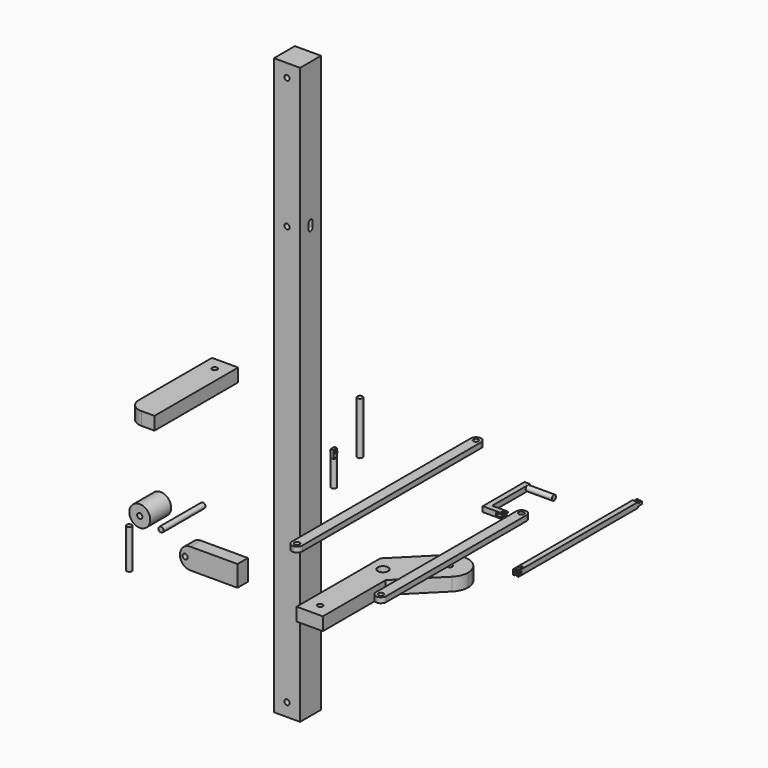
from build123d import *

# Parameters (mm, degrees)
F0_W           = 10
F0_H           = 5
F1_DEPTH       = 40
F2_R           = 5
F3_R           = 1
F4_DEPTH       = 10
F6_DEPTH       = 5
F7_R           = 2
F7_R_2         = 1
F8_DEPTH       = 5.001
F9_R           = 1
F10_DEPTH      = 10
F11_W          = 10
F11_H          = 220
F12_DEPTH      = 10
F13_R          = 1
F14_DEPTH      = 15.1366173212
F15_R          = 1
F16_DEPTH      = 15.1366173212
F17_R          = 1
F18_DEPTH      = 20
F19_W          = 4
F19_H          = 2
F20_DEPTH      = 89.44
F21_R          = 1
F22_DEPTH      = 111.2488439361
F23_R          = 1.99999
F24_W          = 4
F24_H          = 2
F25_DEPTH      = 71.08
F26_R          = 1
F27_DEPTH      = 92.3698075909
F28_R          = 1.99999
F29_W          = 6
F29_H          = 2
F30_DEPTH      = 2
F29_W_2        = 2
F29_H_2        = 57
F31_R          = 1
F32_DEPTH      = 10
F33_R          = 1
F34_DEPTH      = 10
F35_W          = 1
F35_H          = 1.7320508076
F36_DEPTH      = 3
F37_R          = 0.5
F38_DEPTH      = 0.5
F38_DEPTH_BACK = 1.5
F39_W          = 2
F39_H          = 1
F40_DEPTH      = 3
F41_R          = 0.5
F42_DEPTH      = 62.7122059742
F43_W          = 2
F43_H          = 1
F44_DEPTH      = 2
F45_R          = 0.5
F46_DEPTH      = 0.5
F46_DEPTH_BACK = 1.5
F47_W          = 1
F47_H          = 2
F48_DEPTH      = 3
F49_R          = 0.5
F50_DEPTH      = 106.8696667108
F52_DEPTH      = 5
F53_R          = 1
F54_DEPTH      = 76.7775256912
F55_R          = 1
F56_DEPTH      = 20
F57_R          = 4
F57_R_2        = 1
F58_DEPTH      = 10
F60_DEPTH      = 25
F61_R          = 1
F62_DEPTH      = 15


# Not quite as in the source:
# - a fillet or chamfer is up to 0.001 mm smaller than in the source, because OpenCascade refuses the exact size


with BuildPart() as f1:
    # F0 (on Front) → F1 (new body)
    with BuildSketch(Plane.XZ):
        with Locations((-59.1135102832, 41.6379347444)):
            Rectangle(F0_W, F0_H)
    extrude(amount=F1_DEPTH)

    # F2
    f2_edges = [f1.edges().sort_by_distance(p)[0] for p in [
        (-64.11351, -40, 41.637935),
    ]]
    fillet(f2_edges, radius=F2_R)

    # F3 (on face) → F4 (cut)
    with BuildSketch(Plane.XY.offset(44.1379347444)):
        with Locations((-59.1135102832, -5)):
            Circle(F3_R)
    extrude(amount=-F4_DEPTH, mode=Mode.SUBTRACT)


with BuildPart() as f6:
    # F5 (on Top) → F6 (new body)
    with BuildSketch(Plane.XY):
        Polygon((19.0748270126, -21.0775861144), (9.0748270126, -11.0775861144), (9.0748270126, -51.0775861144), (19.0748270126, -51.0775861144), align=None)
        with BuildLine():
            Line((23.2169626363, 3.0645495093), (9.0748270126, -11.0775861144))
            Line((9.0748270126, -11.0775861144), (19.0748270126, -21.0775861144))
            Line((19.0748270126, -21.0775861144), (33.2169626363, -6.9354504907))
            ThreePointArc((33.2169626363, -6.9354504907), (23.2169626363, -6.9354504907), (23.2169626363, 3.0645495093))
        make_face()
        with BuildLine():
            ThreePointArc((35.2880304482, -1.9354504907), (30.9229431371, 4.5973643337), (23.2169626363, 3.0645495093))
            Line((23.2169626363, 3.0645495093), (33.2169626363, -6.9354504907))
            ThreePointArc((33.2169626363, -6.9354504907), (34.7497774607, -4.6414309914), (35.2880304482, -1.9354504907))
        make_face()
        with BuildLine():
            Line((33.2169626363, -6.9354504907), (23.2169626363, 3.0645495093))
            ThreePointArc((23.2169626363, 3.0645495093), (23.2169626363, -6.9354504907), (33.2169626363, -6.9354504907))
        make_face()
    extrude(amount=F6_DEPTH)

    # F7 (on face) → F8 (cut, through all)
    with BuildSketch(Plane.XY.offset(5)):
        with Locations((14.0748270126, -16.0775861144)):
            Circle(F7_R)
        with Locations((28.2169626363, -1.9354504907)):
            Circle(F7_R_2)
    extrude(amount=-F8_DEPTH, mode=Mode.SUBTRACT)

    # F9 (on face) → F10 (cut)
    with BuildSketch(Plane.XY.offset(5)):
        with Locations((14.0748270126, -46.0775861144)):
            Circle(F9_R)
    extrude(amount=-F10_DEPTH, mode=Mode.SUBTRACT)


with BuildPart() as f12:
    # F11 (on Front) → F12 (new body)
    with BuildSketch(Plane.XZ):
        with Locations((-27.4568982422, 49.2887940258)):
            Rectangle(F11_W, F11_H)
    extrude(amount=F12_DEPTH)

    # F13 (on face) → F14 (cut, through all)
    with BuildSketch(Plane.XZ.offset(10)):
        with Locations((-27.4568982422, 154.2887940258)):
            Circle(F13_R)
        with Locations((-27.4568982422, 104.2887940258)):
            Circle(F13_R)
    extrude(amount=-F14_DEPTH, mode=Mode.SUBTRACT)

    # F15 (on face) → F16 (cut, through all)
    with BuildSketch(Plane.XZ.offset(10)):
        with Locations((-27.4568982422, -55.7112059742)):
            Circle(F15_R)
    extrude(amount=-F16_DEPTH, mode=Mode.SUBTRACT)

    # F59 (on face) → F60 (cut)
    with BuildSketch(Plane.YZ.offset(-22.4568982422)):
        with BuildLine():
            Line((-4, 103.2887940258), (-4, 105.2887940258))
            ThreePointArc((-4, 105.2887940258), (-5, 106.2887940258), (-6, 105.2887940258))
            Line((-6, 105.2887940258), (-6, 103.2887940258))
            ThreePointArc((-6, 103.2887940258), (-5, 102.2887940258), (-4, 103.2887940258))
        make_face()
    extrude(amount=-F60_DEPTH, mode=Mode.SUBTRACT)


with BuildPart() as f18:
    # F17 (on Top) → F18 (new body)
    with BuildSketch(Plane.XY):
        with Locations((-42.6939688623, 43.9008660614)):
            Circle(F17_R)
    extrude(amount=F18_DEPTH)


with BuildPart() as f20:
    # F19 (on Front) → F20 (new body)
    with BuildSketch(Plane.XZ):
        with Locations((38.3347739237, 49.5366379619)):
            Rectangle(F19_W, F19_H)
    extrude(amount=F20_DEPTH)

    # F21 (on face) → F22 (cut, through all)
    with BuildSketch(Plane.XY.offset(50.5366379619)):
        with Locations((38.3347739237, -2)):
            Circle(F21_R)
        with Locations((38.3347739237, -87.44)):
            Circle(F21_R)
    extrude(amount=-F22_DEPTH, mode=Mode.SUBTRACT)

    # F23 (radius 2 in the source; OpenCascade refuses exactly that, so slightly less here)
    f23_edges = [f20.edges().sort_by_distance(p)[0] for p in [
        (36.334774, -89.44, 49.536638),
        (40.334774, -89.44, 49.536638),
        (40.334774, 0, 49.536638),
        (36.334774, 0, 49.536638),
    ]]
    fillet(f23_edges, radius=F23_R)


with BuildPart() as f25:
    # F24 (on Front) → F25 (new body)
    with BuildSketch(Plane.XZ):
        with Locations((55.6969568133, 30.6576016166)):
            Rectangle(F24_W, F24_H)
    extrude(amount=F25_DEPTH)

    # F26 (on face) → F27 (cut, through all)
    with BuildSketch(Plane.XY.offset(31.6576016166)):
        with Locations((55.6969568133, -2)):
            Circle(F26_R)
        with Locations((55.6969568133, -69.08)):
            Circle(F26_R)
    extrude(amount=-F27_DEPTH, mode=Mode.SUBTRACT)

    # F28 (radius 2 in the source; OpenCascade refuses exactly that, so slightly less here)
    f28_edges = [f25.edges().sort_by_distance(p)[0] for p in [
        (57.696957, 0, 30.657602),
        (53.696957, 0, 30.657602),
        (57.696957, -71.08, 30.657602),
        (53.696957, -71.08, 30.657602),
    ]]
    fillet(f28_edges, radius=F28_R)


with BuildPart() as f30:
    # F29 (on Top) → F30 (new body)
    with BuildSketch(Plane.XY):
        Polygon((10.2594563812, 58.8238169253), (8.2594563812, 58.8238169253), (8.2594563812, 38.8238169253), (10.2594563812, 38.8238169253), (10.2594563812, 40.8238169253), align=None)
        with Locations((13.2594563812, 39.8238169253)):
            Rectangle(F29_W, F29_H)
    extrude(amount=F30_DEPTH)

    # F31 (on face) → F32 (join)
    with BuildSketch(Plane.YZ.offset(10.2594563812)):
        with Locations((57.8238169253, 1)):
            Circle(F31_R)
    extrude(amount=F32_DEPTH)

    # F39 (on face) → F40 (cut)
    with BuildSketch(Plane.YZ.offset(16.2594563812)):
        with Locations((39.8238169253, 1)):
            Rectangle(F39_W, F39_H)
    extrude(amount=-F40_DEPTH, mode=Mode.SUBTRACT)

    # F41 (on face) → F42 (cut, through all)
    with BuildSketch(Plane.XY.offset(2)):
        with Locations((15.2594563812, 39.8238169253)):
            Circle(F41_R)
    extrude(amount=-F42_DEPTH, mode=Mode.SUBTRACT)


with BuildPart() as f30b:
    # F29 (on Top) → F30, piece 2 (new body)
    with BuildSketch(Plane.XY):
        with Locations((41.7551564276, 41.2765256912)):
            Rectangle(F29_W_2, F29_H_2)
    extrude(amount=F30_DEPTH)

    # F43 (on face) → F44 (join)
    with BuildSketch(Plane(origin=(0, 69.7765256912, 0), x_dir=(-1, 0, 0), z_dir=(0, 1, 0))):
        with Locations((-41.7551564276, 1)):
            Rectangle(F43_W, F43_H)
    extrude(amount=F44_DEPTH)

    # F45 (on face) → F46 (join, two sides)
    with BuildSketch(Plane(origin=(0, 0, 0.5), x_dir=(1, 0, 0), z_dir=(0, 0, -1))) as f46_sk:
        with Locations((41.7551564276, -70.7765256912)):
            Circle(F45_R)
    extrude(amount=F46_DEPTH)
    extrude(f46_sk.sketch, amount=-F46_DEPTH_BACK)

    # F47 (on face) → F48 (cut)
    with BuildSketch(Plane.XZ.offset(-12.7765256912)):
        with Locations((41.7551564276, 1)):
            Rectangle(F47_W, F47_H)
    extrude(amount=-F48_DEPTH, mode=Mode.SUBTRACT)

    # F49 (on face) → F50 (cut, through all)
    with BuildSketch(Plane.YZ.offset(42.7551564276)):
        with Locations((13.7765256912, 1)):
            Circle(F49_R)
    extrude(amount=-F50_DEPTH, mode=Mode.SUBTRACT)


with BuildPart() as f34:
    # F33 (on Top) → F34 (new body)
    with BuildSketch(Plane.XY):
        with Locations((-36.5500971675, 23.7070061266)):
            Circle(F33_R)
    extrude(amount=F34_DEPTH)

    # F35 (on face) → F36 (join)
    with BuildSketch(Plane.XY.offset(10)):
        with Locations((-36.5500971675, 23.7070061266)):
            Rectangle(F35_W, F35_H)
    extrude(amount=F36_DEPTH)

    # F37 (on face) → F38 (join, two sides)
    with BuildSketch(Plane(origin=(-37.0500971675, 0, 0), x_dir=(0, -1, 0), z_dir=(-1, 0, 0))) as f38_sk:
        with Locations((-23.7070061266, 12)):
            Circle(F37_R)
    extrude(amount=F38_DEPTH)
    extrude(f38_sk.sketch, amount=-F38_DEPTH_BACK)


with BuildPart() as f52:
    # F51 (on Front) → F52 (new body)
    with BuildSketch(Plane.XZ):
        with BuildLine():
            Line((-50.3818303212, -18.7227926478), (-68.3818303212, -18.7227926478))
            ThreePointArc((-68.3818303212, -18.7227926478), (-72.3818303212, -22.7227926478), (-68.3818303212, -26.7227926478))
            Line((-68.3818303212, -26.7227926478), (-50.3818303212, -26.7227926478))
            Line((-50.3818303212, -26.7227926478), (-50.3818303212, -18.7227926478))
        make_face()
    extrude(amount=F52_DEPTH)

    # F53 (on face) → F54 (cut, through all)
    with BuildSketch(Plane.XZ.offset(5)):
        with Locations((-70.3818303212, -22.7227926478)):
            Circle(F53_R)
    extrude(amount=-F54_DEPTH, mode=Mode.SUBTRACT)


with BuildPart() as f56:
    # F55 (on Front) → F56 (new body)
    with BuildSketch(Plane.XZ):
        with Locations((-67.6065161824, -6.6479626112)):
            Circle(F55_R)
    extrude(amount=F56_DEPTH)


with BuildPart() as f58:
    # F57 (on Front) → F58 (new body)
    with BuildSketch(Plane.XZ):
        with Locations((-83.7295502424, -11.3588469103)):
            Circle(F57_R)
        with Locations((-83.7295502424, -11.3588469103)):
            Circle(F57_R_2, mode=Mode.SUBTRACT)
    extrude(amount=F58_DEPTH)


with BuildPart() as f62:
    # F61 (on Top) → F62 (new body)
    with BuildSketch(Plane.XY):
        with Locations((-50.596781075, -56.3872568309)):
            Circle(F61_R)
    extrude(amount=F62_DEPTH)


solid = Compound([f1.part, f6.part, f12.part, f18.part, f20.part, f25.part, f30.part, f30b.part, f34.part, f52.part, f56.part, f58.part, f62.part])
